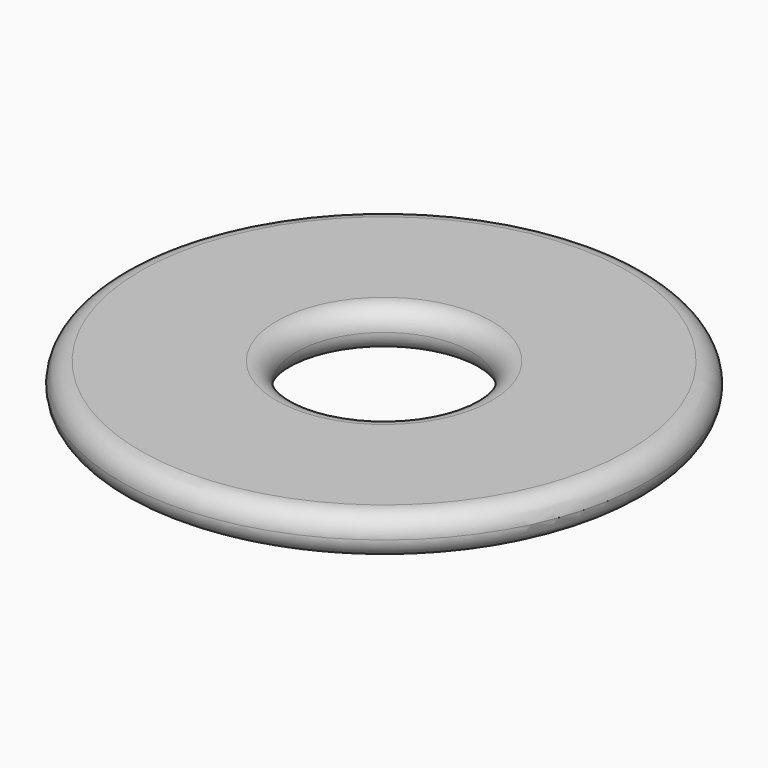
from build123d import *

# Parameters (mm, degrees)
F0_R     = 6.5
F0_R_2   = 2.15
F1_DEPTH = 1
F2_R     = 0.49999


# Not quite as in the source:
# - a fillet or chamfer is up to 0.001 mm smaller than in the source, because OpenCascade refuses the exact size


with BuildPart() as f1:
    # F0 (on Top) → F1 (new body)
    with BuildSketch(Plane.XY):
        Circle(F0_R)
        Circle(F0_R_2, mode=Mode.SUBTRACT)
    extrude(amount=F1_DEPTH)

    # F2 (radius 0.5 in the source; OpenCascade refuses exactly that, so slightly less here)
    f2_edges = [f1.edges().sort_by_distance(p)[0] for p in [
        (-6.5, 0, 1),
        (-2.15, 0, 1),
        (6.5, 0, 0.5),
        (-6.5, 0, 0),
        (-2.15, 0, 0),
        (2.15, 0, 0.5),
    ]]
    fillet(f2_edges, radius=F2_R)


solid = f1.part
